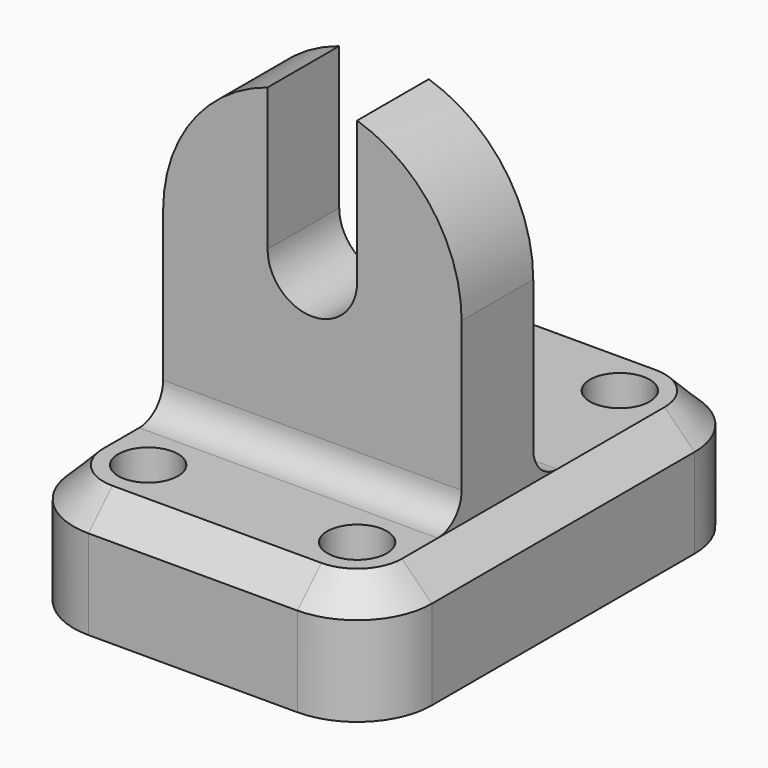
from build123d import *

# Parameters (mm, degrees)
F1_DEPTH = 25.4
F2_SIZE  = 6.35
F3_W     = 63.5
F3_H     = 19.05
F4_DEPTH = 95.25
F6_DEPTH = 25.4
F7_DEPTH = 25.4
F8_D     = 12.7
F9_R     = 6.35


with BuildPart() as f1:
    # F0 (on Top) → F1 (new body)
    with BuildSketch(Plane.XY):
        with BuildLine():
            Line((21.3436168045, 42.000080753), (-23.1063831955, 42.000080753))
            ThreePointArc((-23.1063831955, 42.000080753), (-34.3317033469, 37.3504009043), (-38.9813831955, 26.125080753))
            Line((-38.9813831955, 26.125080753), (-38.9813831955, -43.724919247))
            ThreePointArc((-38.9813831955, -43.724919247), (-34.3317033469, -54.9502393984), (-23.1063831955, -59.599919247))
            Line((-23.1063831955, -59.599919247), (21.3436168045, -59.599919247))
            ThreePointArc((21.3436168045, -59.599919247), (32.5689369558, -54.9502393984), (37.2186168045, -43.724919247))
            Line((37.2186168045, -43.724919247), (37.2186168045, 26.125080753))
            ThreePointArc((37.2186168045, 26.125080753), (32.5689369558, 37.3504009043), (21.3436168045, 42.000080753))
        make_face()
    extrude(amount=F1_DEPTH)

    # F2
    f2_edges = [f1.edges().sort_by_distance(p)[0] for p in [
        (-0.881383, 42.000081, 25.4),
        (37.218617, -8.799919, 25.4),
        (32.568937, 37.350401, 25.4),
        (-34.331703, 37.350401, 25.4),
        (-38.981383, -8.799919, 25.4),
        (-34.331703, -54.950239, 25.4),
        (-0.881383, -59.599919, 25.4),
        (32.568937, -54.950239, 25.4),
    ]]
    chamfer(f2_edges, length=F2_SIZE)

    # F3 (on face) → F4 (join)
    with BuildSketch(Plane.XY.offset(25.4)):
        with Locations((-0.8813831955, -18.324919247)):
            Rectangle(F3_W, F3_H)
    extrude(amount=F4_DEPTH)

    # F5 (on face) → F6 (cut)
    with BuildSketch(Plane.XZ.offset(27.849919247)):
        with BuildLine():
            ThreePointArc((8.6436168045, 93.787569645), (24.7162851553, 82.2835533113), (30.8686168045, 63.5))
            Line((30.8686168045, 63.5), (30.8686168045, 120.65))
            Line((30.8686168045, 120.65), (-32.6313831955, 120.65))
            Line((-32.6313831955, 120.65), (-32.6313831955, 63.5))
            ThreePointArc((-32.6313831955, 63.5), (-26.4790515464, 82.2835533113), (-10.4063831955, 93.787569645))
            ThreePointArc((-10.4063831955, 93.787569645), (-0.8813831955, 95.25), (8.6436168045, 93.787569645))
        make_face()
    extrude(amount=-F6_DEPTH, mode=Mode.SUBTRACT)

    # F5 (on face) → F7 (cut)
    with BuildSketch(Plane.XZ.offset(27.849919247)):
        with BuildLine():
            ThreePointArc((-10.4063831955, 63.5), (-0.8813831955, 53.975), (8.6436168045, 63.5))
            ThreePointArc((8.6436168045, 63.5), (-0.8813831955, 73.025), (-10.4063831955, 63.5))
        make_face()
        with BuildLine():
            Line((8.6436168045, 63.5), (8.6436168045, 93.787569645))
            ThreePointArc((8.6436168045, 93.787569645), (-0.8813831955, 95.25), (-10.4063831955, 93.787569645))
            Line((-10.4063831955, 93.787569645), (-10.4063831955, 63.5))
            ThreePointArc((-10.4063831955, 63.5), (-0.8813831955, 73.025), (8.6436168045, 63.5))
        make_face()
    extrude(amount=-F7_DEPTH, mode=Mode.SUBTRACT)

    # F8 (through all)
    with Locations(Plane(origin=(0, 0, 0), x_dir=(1, 0, 0), z_dir=(0, 0, -1))):
        with Locations((-23.1063831955, 43.724919247), (21.3436168045, 43.724919247), (-23.1063831955, -26.125080753), (21.3436168045, -26.125080753)):
            Hole(F8_D / 2)

    # F9
    f9_edges = [f1.edges().sort_by_distance(p)[0] for p in [
        (-0.881383, -8.799919, 25.4),
        (-0.881383, -27.849919, 25.4),
    ]]
    fillet(f9_edges, radius=F9_R)


solid = f1.part
